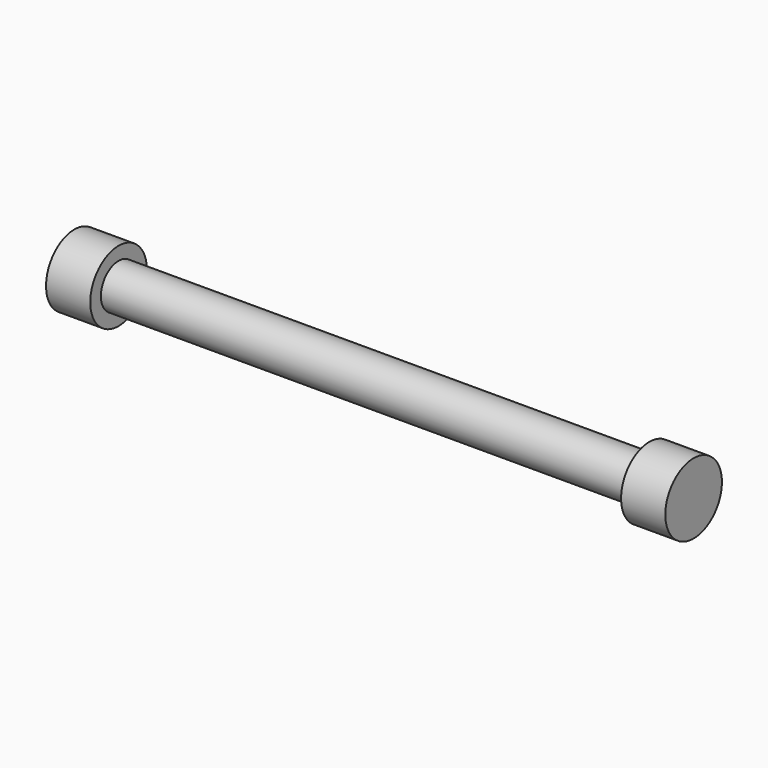
from build123d import *

# Parameters (mm, degrees)
F0_R     = 3.175
F1_DEPTH = 38.1
F2_R     = 5.08
F2_R_2   = 3.175
F3_DEPTH = 6.35


# Not quite as in the source:
# - a pattern or mirror of a feature is missing from the dataset's text; its kind, count and spacing are read off the source's solid


with BuildPart() as f1:
    # F0 (on Right) → F1 (new body, symmetric)
    with BuildSketch(Plane.YZ):
        Circle(F0_R)
    extrude(amount=F1_DEPTH, both=True)

    # F2 (on face) → F3 (join)
    with BuildSketch(Plane.YZ.offset(38.1)):
        Circle(F2_R)
        Circle(F2_R_2, mode=Mode.SUBTRACT)
        Circle(F2_R_2)
    f3 = extrude(amount=F3_DEPTH)

    # F3_copies: F3 across plane
    add(f3.mirror(Plane(origin=(0, 0, 0), x_dir=(0, 0, -1), z_dir=(-1, 0, 0))))


solid = f1.part
